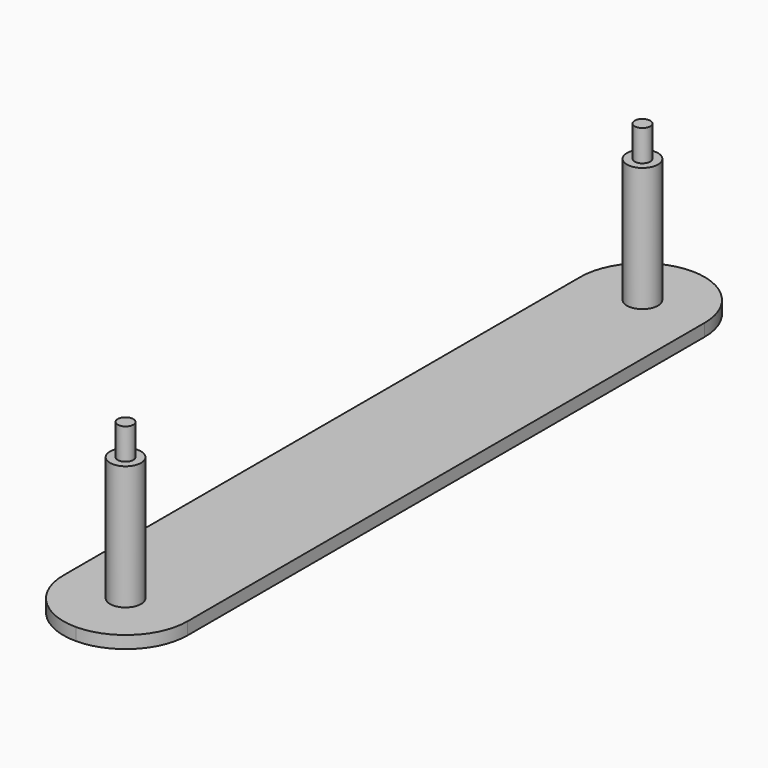
from build123d import *

# Parameters (mm, degrees)
F0_R     = 3.175
F0_R_2   = 1.5875
F1_DEPTH = 2.54
F2_DEPTH = 25.4
F3_R     = 12.69999
F4_DEPTH = 31.75


# Not quite as in the source:
# - a fillet or chamfer is up to 0.001 mm smaller than in the source, because OpenCascade refuses the exact size


with BuildPart() as f1:
    # F0 (on Top) → F1 (new body)
    with BuildSketch(Plane.XY):
        Polygon((12.7, 144.78), (0, 144.78), (-12.7, 144.78), (-12.7, -12.7), (0, -12.7), (12.7, -12.7), align=None)
        Circle(F0_R, mode=Mode.SUBTRACT)
        with Locations((0, 132.08)):
            Circle(F0_R, mode=Mode.SUBTRACT)
        with Locations((0, 132.08)):
            Circle(F0_R)
        with Locations((0, 132.08)):
            Circle(F0_R_2, mode=Mode.SUBTRACT)
        with Locations((0, 132.08)):
            Circle(F0_R_2)
        Circle(F0_R)
        Circle(F0_R_2, mode=Mode.SUBTRACT)
        Circle(F0_R_2)
    extrude(amount=-F1_DEPTH)

    # F0 (on Top) → F2 (join)
    with BuildSketch(Plane.XY):
        with Locations((0, 132.08)):
            Circle(F0_R)
        with Locations((0, 132.08)):
            Circle(F0_R_2, mode=Mode.SUBTRACT)
        Circle(F0_R)
        Circle(F0_R_2, mode=Mode.SUBTRACT)
        with Locations((0, 132.08)):
            Circle(F0_R_2)
        Circle(F0_R_2)
    extrude(amount=F2_DEPTH)

    # F3 (radius 12.7 in the source; OpenCascade refuses exactly that, so slightly less here)
    f3_edges = [f1.edges().sort_by_distance(p)[0] for p in [
        (12.7, 144.78, -1.27),
        (-12.7, 144.78, -1.27),
        (-12.7, -12.7, -1.27),
        (12.7, -12.7, -1.27),
    ]]
    fillet(f3_edges, radius=F3_R)

    # F0 (on Top) → F4 (join)
    with BuildSketch(Plane.XY):
        Circle(F0_R_2)
        with Locations((0, 132.08)):
            Circle(F0_R_2)
    extrude(amount=F4_DEPTH)


solid = f1.part
